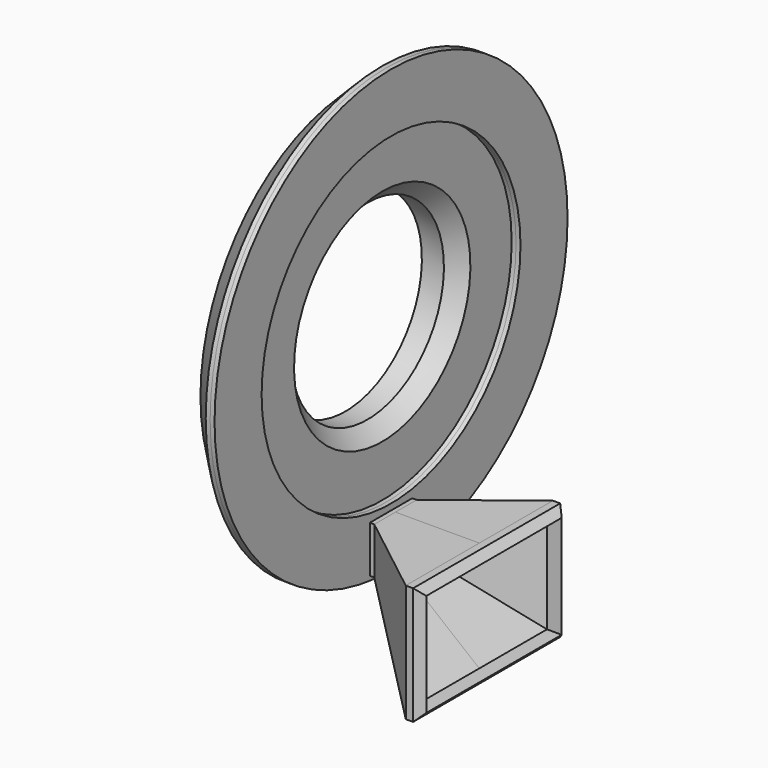
from build123d import *

# Parameters (mm, degrees)
F0_W      = 5
F0_H      = 2.0118219405
F2_SIZE   = 4.99999
F3_SIZE   = 2
F4_SIZE   = 2
F5_R      = 23
F5_R_2    = 22
F6_DEPTH  = 0.6
F5_R_3    = 30
F5_R_4    = 28.4994588965
F7_R      = 30
F7_R_2    = 22
F8_DEPTH  = 0.6
F9_W      = 3.6018721294
F9_H      = 6.3549551666
F10_DEPTH = 0.6
F12_DEPTH = 16
F15_W     = 11.5
F15_H     = 14
F16_DEPTH = 25
F14_W     = 11.5
F14_H     = 14
F13_W     = 3.2251703087
F13_H     = 5.2452619672
F18_DEPTH = 25
F21_SIZE  = 0.99999


# Not quite as in the source:
# - a fillet or chamfer is up to 0.001 mm smaller than in the source, because OpenCascade refuses the exact size


with BuildPart() as f1:
    # F0 (on Front) → F1 (revolve)
    with BuildSketch(Plane.XZ):
        Polygon((-2.5, 30), (-2.5, 16.0713382065), (2.5, 30), align=None)
    revolve(axis=Axis((0, 0, 0), (-1, 0, 0)))

    # F2 (size 5 in the source; OpenCascade refuses exactly that, so slightly less here)
    f2_edges = [f1.edges().sort_by_distance(p)[0] for p in [
        (-2.5, 0, -30),
    ]]
    chamfer(f2_edges, length=F2_SIZE)

    # F4
    f4_edges = [f1.edges().sort_by_distance(p)[0] for p in [
        (-2.5, 0, -25.00001),
    ]]
    chamfer(f4_edges, length=F4_SIZE)

    # F14 (on face) → F17 section 0
    with BuildSketch(Plane(origin=(15.7, 0, 0), x_dir=(0, -1, 0), z_dir=(-1, 0, 0))):
        with Locations((5.75, -30.8225224167)):
            Rectangle(F14_W, F14_H)
    # F13 (on face) → F17 section 1
    with BuildSketch(Plane.YZ.offset(4.3)):
        with Locations((-1.6125851544, -26)):
            Rectangle(F13_W, F13_H)
    loft(mode=Mode.SUBTRACT)


with BuildPart() as f1b:
    # F0 (on Front) → F1, piece 2 (revolve)
    with BuildSketch(Plane.XZ):
        Polygon((2.5, 23), (-2.5, 15), (2.5, 15), align=None)
        with Locations((0, 13.9940890297)):
            Rectangle(F0_W, F0_H)
    revolve(axis=Axis((0, 0, 0), (-1, 0, 0)))

    # F3
    f3_edges = [f1b.edges().sort_by_distance(p)[0] for p in [
        (2.5, 0, -12.988178),
    ]]
    chamfer(f3_edges, length=F3_SIZE)

    # F5 (on face) → F6 (join)
    with BuildSketch(Plane.YZ.offset(2.5)):
        Circle(F5_R)
        Circle(F5_R_2, mode=Mode.SUBTRACT)
    extrude(amount=F6_DEPTH)


with BuildPart() as f6:
    # F5 (on face) → F6, piece 2 (new body)
    with BuildSketch(Plane.YZ.offset(2.5)):
        Circle(F5_R_3)
        Circle(F5_R_4, mode=Mode.SUBTRACT)
    extrude(amount=F6_DEPTH)


with BuildPart() as f8:
    # F7 (on face) → F8 (new body)
    with BuildSketch(Plane.YZ.offset(3.1)):
        Circle(F7_R)
        Circle(F7_R_2, mode=Mode.SUBTRACT)
    extrude(amount=F8_DEPTH)

    # F9 (on face) → F10 (join)
    with BuildSketch(Plane.YZ.offset(3.7)):
        with Locations((-1.8009360647, -26)):
            Rectangle(F9_W, F9_H)
        with Locations((1.8009360647, -26)):
            Rectangle(F9_W, F9_H)
    extrude(amount=F10_DEPTH)


with BuildPart() as f12:
    # F11 (on face) → F12 (new body)
    with BuildSketch(Plane.XY.offset(-22.8225224167)):
        Polygon((15.7, -6.078068167), (17.4430608749, -6.078068167), (17.4430608749, 12.5), (15.7, 12.5), (15.7, 0), align=None)
        Polygon((17.4430608749, 12.5), (17.4430608749, -6.078068167), (15.7, -6.078068167), (15.7, -12.5), (17.7, -12.5), (17.7, 12.5), align=None)
    extrude(amount=-F12_DEPTH)

    # F15 (on face) → F16 (cut)
    with BuildSketch(Plane.YZ.offset(17.7)):
        with Locations((5.75, -30.8225224167)):
            Rectangle(F15_W, F15_H)
        with Locations((-5.75, -30.8225224167)):
            Rectangle(F15_W, F15_H)
    extrude(amount=-F16_DEPTH, mode=Mode.SUBTRACT)

    # F21 (size 1 in the source; OpenCascade refuses exactly that, so slightly less here)
    f21_edges = [f12.edges().sort_by_distance(p)[0] for p in [
        (17.7, 0, -22.822522),
        (17.7, 0, -38.822522),
        (17.7, -12.5, -30.822522),
        (17.7, 12.5, -30.822522),
    ]]
    chamfer(f21_edges, length=F21_SIZE)


with BuildPart() as f18_tool:
    # F13 (on face) → F18 (new body)
    with BuildSketch(Plane.YZ.offset(4.3)):
        with Locations((-1.6125851544, -26)):
            Rectangle(F13_W, F13_H)
        with Locations((1.6125851544, -26)):
            Rectangle(F13_W, F13_H)
    extrude(amount=-F18_DEPTH)


with BuildPart() as f6_1:
    add(f6.part)

    # F18: cut by f18_tool
    add(f18_tool.part, mode=Mode.SUBTRACT)


with BuildPart() as f8_1:
    add(f8.part)

    # F18: cut by f18_tool
    add(f18_tool.part, mode=Mode.SUBTRACT)


with BuildPart() as f19:
    # F13 (on face) → F19 section 0
    with BuildSketch(Plane.YZ.offset(4.3)):
        Polygon((0, -23.3773690164), (0, -22.8225224167), (-3.6018721294, -22.8225224167), (-3.6018721294, -29.1774775833), (0, -29.1774775833), (0, -28.6226309836), (-3.2251703087, -28.6226309836), (-3.2251703087, -23.3773690164), align=None)
    # F14 (on face) → F19 section 1
    with BuildSketch(Plane(origin=(15.7, 0, 0), x_dir=(0, -1, 0), z_dir=(-1, 0, 0))):
        Polygon((0, -37.8225224167), (0, -38.8225224167), (12.5, -38.8225224167), (12.5, -22.8225224167), (0, -22.8225224167), (0, -23.8225224167), (11.5, -23.8225224167), (11.5, -37.8225224167), align=None)
    loft()


with BuildPart() as f20:
    # F13 (on face) → F20 section 0
    with BuildSketch(Plane.YZ.offset(4.3)):
        Polygon((3.6018721294, -22.8225224167), (0, -22.8225224167), (0, -23.3773690164), (3.2251703087, -23.3773690164), (3.2251703087, -28.6226309836), (0, -28.6226309836), (0, -29.1774775833), (3.6018721294, -29.1774775833), align=None)
    # F14 (on face) → F20 section 1
    with BuildSketch(Plane(origin=(15.7, 0, 0), x_dir=(0, -1, 0), z_dir=(-1, 0, 0))):
        Polygon((-12.5, -38.8225224167), (0, -38.8225224167), (0, -37.8225224167), (-11.5, -37.8225224167), (-11.5, -23.8225224167), (0, -23.8225224167), (0, -22.8225224167), (-12.5, -22.8225224167), align=None)
    loft()


solid = Compound([f1.part, f1b.part, f12.part, f6_1.part, f8_1.part, f19.part, f20.part])
